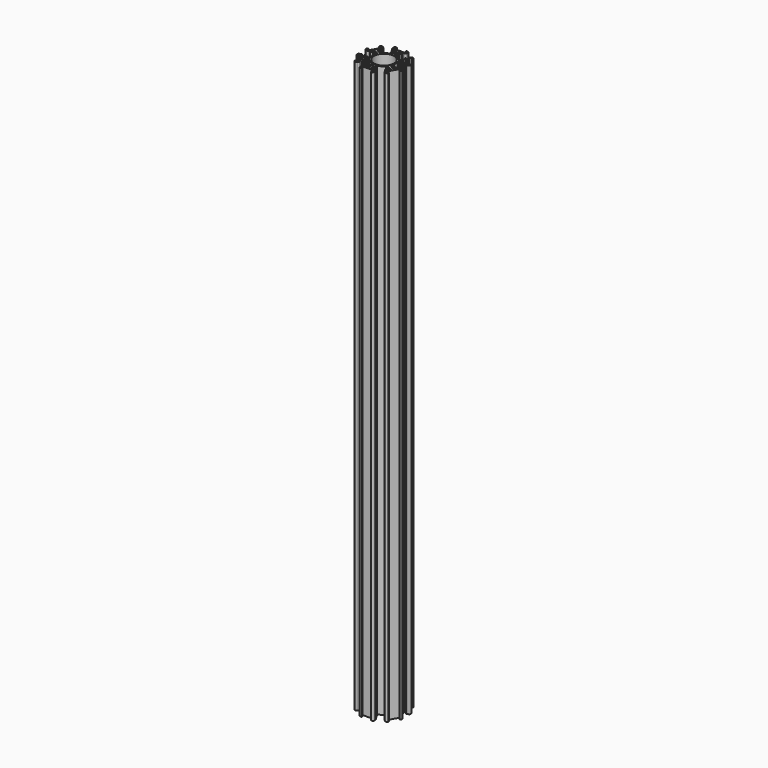
from build123d import *

# Parameters (mm, degrees)
F0_R     = 10.5
F1_DEPTH = 600
F2_R     = 1.5
F3_R     = 0.49999
F4_R     = 0.5
F6_DEPTH = 600.001
F7_R     = 0.5
F8_R     = 1.5


# Not quite as in the source:
# - a fillet or chamfer is up to 0.001 mm smaller than in the source, because OpenCascade refuses the exact size


with BuildPart() as f1:
    # F0 (on Top) → F1 (new body)
    with BuildSketch(Plane.XY):
        with BuildLine():
            Line((-7.45, -19.1599357944), (-7.45, -23.5599357944))
            Line((-7.45, -23.5599357944), (-4.75, -23.5599357944))
            Line((-4.75, -23.5599357944), (-4.75, -22.3599357944))
            Line((-4.75, -22.3599357944), (-6.25, -22.3599357944))
            Line((-6.25, -22.3599357944), (-6.25, -20.3599357944))
            Line((-6.25, -20.3599357944), (6.25, -20.3599357944))
            Line((6.25, -20.3599357944), (6.25, -22.3599357944))
            Line((6.25, -22.3599357944), (4.75, -22.3599357944))
            Line((4.75, -22.3599357944), (4.75, -23.5599357944))
            Line((4.75, -23.5599357944), (7.45, -23.5599357944))
            Line((7.45, -23.5599357944), (7.45, -19.1599357944))
            Line((7.45, -19.1599357944), (1, -19.1599357944))
            Line((1, -19.1599357944), (1, -17.4599357944))
            Line((1, -17.4599357944), (5.5, -17.4599357944))
            Line((5.5, -17.4599357944), (5.5, -16.4599357944))
            Line((5.5, -16.4599357944), (1, -16.4599357944))
            Line((1, -16.4599357944), (1, -14.8599357944))
            Line((1, -14.8599357944), (4, -14.8599357944))
            Line((4, -14.8599357944), (4, -13.8599357944))
            Line((4, -13.8599357944), (1, -13.8599357944))
            Line((1, -13.8599357944), (1, -12.4599357944))
            ThreePointArc((1, -12.4599357944), (6.25, -10.8253175473), (10.2906209275, -7.095993301))
            Line((10.2906209275, -7.095993301), (11.5030564928, -7.795993301))
            Line((11.5030564928, -7.795993301), (10.0030564928, -10.3940695123))
            Line((10.0030564928, -10.3940695123), (10.8690818965, -10.8940695123))
            Line((10.8690818965, -10.8940695123), (12.3690818965, -8.295993301))
            Line((12.3690818965, -8.295993301), (13.7547225426, -9.095993301))
            Line((13.7547225426, -9.095993301), (11.5047225426, -12.993107618))
            Line((11.5047225426, -12.993107618), (12.3707479464, -13.493107618))
            Line((12.3707479464, -13.493107618), (14.6207479464, -9.595993301))
            Line((14.6207479464, -9.595993301), (16.0929911328, -10.445993301))
            Line((16.0929911328, -10.445993301), (12.8679911328, -16.0318571554))
            Line((12.8679911328, -16.0318571554), (16.6785029095, -18.2318571554))
            Line((16.6785029095, -18.2318571554), (18.0285029095, -15.8935885652))
            Line((18.0285029095, -15.8935885652), (16.9892724249, -15.2935885652))
            Line((16.9892724249, -15.2935885652), (16.2392724249, -16.5926266708))
            Line((16.2392724249, -16.5926266708), (14.5072216174, -15.5926266708))
            Line((14.5072216174, -15.5926266708), (20.7572216174, -4.7673091235))
            Line((20.7572216174, -4.7673091235), (22.4892724249, -5.7673091235))
            Line((22.4892724249, -5.7673091235), (21.7392724249, -7.0663472292))
            Line((21.7392724249, -7.0663472292), (22.7785029095, -7.6663472292))
            Line((22.7785029095, -7.6663472292), (24.1285029095, -5.328078639))
            Line((24.1285029095, -5.328078639), (20.3179911328, -3.128078639))
            Line((20.3179911328, -3.128078639), (17.0929911328, -8.7139424934))
            Line((17.0929911328, -8.7139424934), (15.6207479464, -7.8639424934))
            Line((15.6207479464, -7.8639424934), (17.8707479464, -3.9668281764))
            Line((17.8707479464, -3.9668281764), (17.0047225426, -3.4668281764))
            Line((17.0047225426, -3.4668281764), (14.7547225426, -7.3639424934))
            Line((14.7547225426, -7.3639424934), (13.3690818965, -6.5639424934))
            Line((13.3690818965, -6.5639424934), (14.8690818965, -3.9658662821))
            Line((14.8690818965, -3.9658662821), (14.0030564928, -3.4658662821))
            Line((14.0030564928, -3.4658662821), (12.5030564928, -6.0639424934))
            Line((12.5030564928, -6.0639424934), (11.2906209275, -5.3639424934))
            ThreePointArc((11.2906209275, -5.3639424934), (12.5, 0), (11.2906209275, 5.3639424934))
            Line((11.2906209275, 5.3639424934), (12.5030564928, 6.0639424934))
            Line((12.5030564928, 6.0639424934), (14.0030564928, 3.4658662821))
            Line((14.0030564928, 3.4658662821), (14.8690818965, 3.9658662821))
            Line((14.8690818965, 3.9658662821), (13.3690818965, 6.5639424934))
            Line((13.3690818965, 6.5639424934), (14.7547225426, 7.3639424934))
            Line((14.7547225426, 7.3639424934), (17.0047225426, 3.4668281764))
            Line((17.0047225426, 3.4668281764), (17.8707479464, 3.9668281764))
            Line((17.8707479464, 3.9668281764), (15.6207479464, 7.8639424934))
            Line((15.6207479464, 7.8639424934), (17.0929911328, 8.7139424934))
            Line((17.0929911328, 8.7139424934), (20.3179911328, 3.128078639))
            Line((20.3179911328, 3.128078639), (24.1285029095, 5.328078639))
            Line((24.1285029095, 5.328078639), (22.7785029095, 7.6663472292))
            Line((22.7785029095, 7.6663472292), (21.7392724249, 7.0663472292))
            Line((21.7392724249, 7.0663472292), (22.4892724249, 5.7673091235))
            Line((22.4892724249, 5.7673091235), (20.7572216174, 4.7673091235))
            Line((20.7572216174, 4.7673091235), (14.5072216174, 15.5926266708))
            Line((14.5072216174, 15.5926266708), (16.2392724249, 16.5926266708))
            Line((16.2392724249, 16.5926266708), (16.9892724249, 15.2935885652))
            Line((16.9892724249, 15.2935885652), (18.0285029095, 15.8935885652))
            Line((18.0285029095, 15.8935885652), (16.6785029095, 18.2318571554))
            Line((16.6785029095, 18.2318571554), (12.8679911328, 16.0318571554))
            Line((12.8679911328, 16.0318571554), (16.0929911328, 10.445993301))
            Line((16.0929911328, 10.445993301), (14.6207479464, 9.595993301))
            Line((14.6207479464, 9.595993301), (12.3707479464, 13.493107618))
            Line((12.3707479464, 13.493107618), (11.5047225426, 12.993107618))
            Line((11.5047225426, 12.993107618), (13.7547225426, 9.095993301))
            Line((13.7547225426, 9.095993301), (12.3690818965, 8.295993301))
            Line((12.3690818965, 8.295993301), (10.8690818965, 10.8940695123))
            Line((10.8690818965, 10.8940695123), (10.0030564928, 10.3940695123))
            Line((10.0030564928, 10.3940695123), (11.5030564928, 7.795993301))
            Line((11.5030564928, 7.795993301), (10.2906209275, 7.095993301))
            ThreePointArc((10.2906209275, 7.095993301), (6.25, 10.8253175473), (1, 12.4599357944))
            Line((1, 12.4599357944), (1, 13.8599357944))
            Line((1, 13.8599357944), (4, 13.8599357944))
            Line((4, 13.8599357944), (4, 14.8599357944))
            Line((4, 14.8599357944), (1, 14.8599357944))
            Line((1, 14.8599357944), (1, 16.4599357944))
            Line((1, 16.4599357944), (5.5, 16.4599357944))
            Line((5.5, 16.4599357944), (5.5, 17.4599357944))
            Line((5.5, 17.4599357944), (1, 17.4599357944))
            Line((1, 17.4599357944), (1, 19.1599357944))
            Line((1, 19.1599357944), (7.45, 19.1599357944))
            Line((7.45, 19.1599357944), (7.45, 23.5599357944))
            Line((7.45, 23.5599357944), (4.75, 23.5599357944))
            Line((4.75, 23.5599357944), (4.75, 22.3599357944))
            Line((4.75, 22.3599357944), (6.25, 22.3599357944))
            Line((6.25, 22.3599357944), (6.25, 20.3599357944))
            Line((6.25, 20.3599357944), (-6.25, 20.3599357944))
            Line((-6.25, 20.3599357944), (-6.25, 22.3599357944))
            Line((-6.25, 22.3599357944), (-4.75, 22.3599357944))
            Line((-4.75, 22.3599357944), (-4.75, 23.5599357944))
            Line((-4.75, 23.5599357944), (-7.45, 23.5599357944))
            Line((-7.45, 23.5599357944), (-7.45, 19.1599357944))
            Line((-7.45, 19.1599357944), (-1, 19.1599357944))
            Line((-1, 19.1599357944), (-1, 17.4599357944))
            Line((-1, 17.4599357944), (-5.5, 17.4599357944))
            Line((-5.5, 17.4599357944), (-5.5, 16.4599357944))
            Line((-5.5, 16.4599357944), (-1, 16.4599357944))
            Line((-1, 16.4599357944), (-1, 14.8599357944))
            Line((-1, 14.8599357944), (-4, 14.8599357944))
            Line((-4, 14.8599357944), (-4, 13.8599357944))
            Line((-4, 13.8599357944), (-1, 13.8599357944))
            Line((-1, 13.8599357944), (-1, 12.4599357944))
            ThreePointArc((-1, 12.4599357944), (-6.25, 10.8253175473), (-10.2906209275, 7.095993301))
            Line((-10.2906209275, 7.095993301), (-11.5030564928, 7.795993301))
            Line((-11.5030564928, 7.795993301), (-10.0030564928, 10.3940695123))
            Line((-10.0030564928, 10.3940695123), (-10.8690818965, 10.8940695123))
            Line((-10.8690818965, 10.8940695123), (-12.3690818965, 8.295993301))
            Line((-12.3690818965, 8.295993301), (-13.7547225426, 9.095993301))
            Line((-13.7547225426, 9.095993301), (-11.5047225426, 12.993107618))
            Line((-11.5047225426, 12.993107618), (-12.3707479464, 13.493107618))
            Line((-12.3707479464, 13.493107618), (-14.6207479464, 9.595993301))
            Line((-14.6207479464, 9.595993301), (-16.0929911328, 10.445993301))
            Line((-16.0929911328, 10.445993301), (-12.8679911328, 16.0318571554))
            Line((-12.8679911328, 16.0318571554), (-16.6785029095, 18.2318571554))
            Line((-16.6785029095, 18.2318571554), (-18.0285029095, 15.8935885652))
            Line((-18.0285029095, 15.8935885652), (-16.9892724249, 15.2935885652))
            Line((-16.9892724249, 15.2935885652), (-16.2392724249, 16.5926266708))
            Line((-16.2392724249, 16.5926266708), (-14.5072216174, 15.5926266708))
            Line((-14.5072216174, 15.5926266708), (-20.7572216174, 4.7673091235))
            Line((-20.7572216174, 4.7673091235), (-22.4892724249, 5.7673091235))
            Line((-22.4892724249, 5.7673091235), (-21.7392724249, 7.0663472292))
            Line((-21.7392724249, 7.0663472292), (-22.7785029095, 7.6663472292))
            Line((-22.7785029095, 7.6663472292), (-24.1285029095, 5.328078639))
            Line((-24.1285029095, 5.328078639), (-20.3179911328, 3.128078639))
            Line((-20.3179911328, 3.128078639), (-17.0929911328, 8.7139424934))
            Line((-17.0929911328, 8.7139424934), (-15.6207479464, 7.8639424934))
            Line((-15.6207479464, 7.8639424934), (-17.8707479464, 3.9668281764))
            Line((-17.8707479464, 3.9668281764), (-17.0047225426, 3.4668281764))
            Line((-17.0047225426, 3.4668281764), (-14.7547225426, 7.3639424934))
            Line((-14.7547225426, 7.3639424934), (-13.3690818965, 6.5639424934))
            Line((-13.3690818965, 6.5639424934), (-14.8690818965, 3.9658662821))
            Line((-14.8690818965, 3.9658662821), (-14.0030564928, 3.4658662821))
            Line((-14.0030564928, 3.4658662821), (-12.5030564928, 6.0639424934))
            Line((-12.5030564928, 6.0639424934), (-11.2906209275, 5.3639424934))
            ThreePointArc((-11.2906209275, 5.3639424934), (-12.5, 0), (-11.2906209275, -5.3639424934))
            Line((-11.2906209275, -5.3639424934), (-12.5030564928, -6.0639424934))
            Line((-12.5030564928, -6.0639424934), (-14.0030564928, -3.4658662821))
            Line((-14.0030564928, -3.4658662821), (-14.8690818965, -3.9658662821))
            Line((-14.8690818965, -3.9658662821), (-13.3690818965, -6.5639424934))
            Line((-13.3690818965, -6.5639424934), (-14.7547225426, -7.3639424934))
            Line((-14.7547225426, -7.3639424934), (-17.0047225426, -3.4668281764))
            Line((-17.0047225426, -3.4668281764), (-17.8707479464, -3.9668281764))
            Line((-17.8707479464, -3.9668281764), (-15.6207479464, -7.8639424934))
            Line((-15.6207479464, -7.8639424934), (-17.0929911328, -8.7139424934))
            Line((-17.0929911328, -8.7139424934), (-20.3179911328, -3.128078639))
            Line((-20.3179911328, -3.128078639), (-24.1285029095, -5.328078639))
            Line((-24.1285029095, -5.328078639), (-22.7785029095, -7.6663472292))
            Line((-22.7785029095, -7.6663472292), (-21.7392724249, -7.0663472292))
            Line((-21.7392724249, -7.0663472292), (-22.4892724249, -5.7673091235))
            Line((-22.4892724249, -5.7673091235), (-20.7572216174, -4.7673091235))
            Line((-20.7572216174, -4.7673091235), (-14.5072216174, -15.5926266708))
            Line((-14.5072216174, -15.5926266708), (-16.2392724249, -16.5926266708))
            Line((-16.2392724249, -16.5926266708), (-16.9892724249, -15.2935885652))
            Line((-16.9892724249, -15.2935885652), (-18.0285029095, -15.8935885652))
            Line((-18.0285029095, -15.8935885652), (-16.6785029095, -18.2318571554))
            Line((-16.6785029095, -18.2318571554), (-12.8679911328, -16.0318571554))
            Line((-12.8679911328, -16.0318571554), (-16.0929911328, -10.445993301))
            Line((-16.0929911328, -10.445993301), (-14.6207479464, -9.595993301))
            Line((-14.6207479464, -9.595993301), (-12.3707479464, -13.493107618))
            Line((-12.3707479464, -13.493107618), (-11.5047225426, -12.993107618))
            Line((-11.5047225426, -12.993107618), (-13.7547225426, -9.095993301))
            Line((-13.7547225426, -9.095993301), (-12.3690818965, -8.295993301))
            Line((-12.3690818965, -8.295993301), (-10.8690818965, -10.8940695123))
            Line((-10.8690818965, -10.8940695123), (-10.0030564928, -10.3940695123))
            Line((-10.0030564928, -10.3940695123), (-11.5030564928, -7.795993301))
            Line((-11.5030564928, -7.795993301), (-10.2906209275, -7.095993301))
            ThreePointArc((-10.2906209275, -7.095993301), (-6.25, -10.8253175473), (-1, -12.4599357944))
            Line((-1, -12.4599357944), (-1, -13.8599357944))
            Line((-1, -13.8599357944), (-4, -13.8599357944))
            Line((-4, -13.8599357944), (-4, -14.8599357944))
            Line((-4, -14.8599357944), (-1, -14.8599357944))
            Line((-1, -14.8599357944), (-1, -16.4599357944))
            Line((-1, -16.4599357944), (-5.5, -16.4599357944))
            Line((-5.5, -16.4599357944), (-5.5, -17.4599357944))
            Line((-5.5, -17.4599357944), (-1, -17.4599357944))
            Line((-1, -17.4599357944), (-1, -19.1599357944))
            Line((-1, -19.1599357944), (-7.45, -19.1599357944))
        make_face()
        Circle(F0_R, mode=Mode.SUBTRACT)
    extrude(amount=F1_DEPTH)

    # F2
    f2_edges = [f1.edges().sort_by_distance(p)[0] for p in [
        (7.45, 19.159936, 300),
        (-7.45, 19.159936, 300),
        (12.867991, 16.031857, 300),
        (20.317991, 3.128079, 300),
        (20.317991, -3.128079, 300),
        (12.867991, -16.031857, 300),
        (7.45, -19.159936, 300),
        (-7.45, -19.159936, 300),
        (-12.867991, -16.031857, 300),
        (-20.317991, -3.128079, 300),
        (-20.317991, 3.128079, 300),
        (-12.867991, 16.031857, 300),
    ]]
    fillet(f2_edges, radius=F2_R)

    # F3 (radius 0.5 in the source; OpenCascade refuses exactly that, so slightly less here)
    f3_edges = [f1.edges().sort_by_distance(p)[0] for p in [
        (4.75, 23.559936, 300),
        (-4.75, 23.559936, 300),
        (-5.5, 17.459936, 300),
        (-5.5, 16.459936, 300),
        (-4, 14.859936, 300),
        (-4, 13.859936, 300),
        (5.5, 17.459936, 300),
        (5.5, 16.459936, 300),
        (4, 14.859936, 300),
        (4, 13.859936, 300),
        (-18.028503, 15.893589, 300),
        (-22.778503, 7.666347, 300),
        (-17.870748, 3.966828, 300),
        (-17.004723, 3.466828, 300),
        (-14.869082, 3.965866, 300),
        (-14.003056, 3.465866, 300),
        (-10.869082, 10.89407, 300),
        (-12.370748, 13.493108, 300),
        (-11.504723, 12.993108, 300),
        (-10.003056, 10.39407, 300),
        (-22.778503, -7.666347, 300),
        (-17.870748, -3.966828, 300),
        (-17.004723, -3.466828, 300),
        (-14.869082, -3.965866, 300),
        (-14.003056, -3.465866, 300),
        (-10.869082, -10.89407, 300),
        (-10.003056, -10.39407, 300),
        (-11.504723, -12.993108, 300),
        (-12.370748, -13.493108, 300),
        (-18.028503, -15.893589, 300),
        (-5.5, -17.459936, 300),
        (-5.5, -16.459936, 300),
        (-4, -14.859936, 300),
        (-4, -13.859936, 300),
        (-4.75, -23.559936, 300),
        (4.75, -23.559936, 300),
        (5.5, -17.459936, 300),
        (5.5, -16.459936, 300),
        (4, -14.859936, 300),
        (4, -13.859936, 300),
        (12.370748, -13.493108, 300),
        (11.504723, -12.993108, 300),
        (10.003056, -10.39407, 300),
        (10.869082, -10.89407, 300),
        (18.028503, -15.893589, 300),
        (22.778503, -7.666347, 300),
        (17.870748, -3.966828, 300),
        (14.869082, -3.965866, 300),
        (17.004723, -3.466828, 300),
        (14.003056, -3.465866, 300),
        (17.004723, 3.466828, 300),
        (17.870748, 3.966828, 300),
        (14.869082, 3.965866, 300),
        (14.003056, 3.465866, 300),
        (10.003056, 10.39407, 300),
        (11.504723, 12.993108, 300),
        (18.028503, 15.893589, 300),
        (22.778503, 7.666347, 300),
        (12.370748, 13.493108, 300),
        (10.869082, 10.89407, 300),
    ]]
    fillet(f3_edges, radius=F3_R)

    # F4
    f4_edges = [f1.edges().sort_by_distance(p)[0] for p in [
        (16.092991, -10.445993, 300),
        (17.092991, -8.713942, 300),
        (-1, -19.159936, 300),
        (1, -19.159936, 300),
        (-16.092991, -10.445993, 300),
        (-17.092991, -8.713942, 300),
        (-17.092991, 8.713942, 300),
        (-16.092991, 10.445993, 300),
        (-1, 19.159936, 300),
        (1, 19.159936, 300),
        (16.092991, 10.445993, 300),
        (17.092991, 8.713942, 300),
    ]]
    fillet(f4_edges, radius=F4_R)

    # F5 (on face) → F6 (cut, through all)
    with BuildSketch(Plane.XY.offset(600)):
        with BuildLine():
            Line((-1, 11.9582604777), (-1, 12.4599357944))
            ThreePointArc((-1, 12.4599357944), (-6.25, 10.8253175473), (-10.2906209275, 7.095993301))
            Line((-10.2906209275, 7.095993301), (-9.8561573587, 6.8451556426))
            ThreePointArc((-9.8561573587, 6.8451556426), (-5.9999998677, 10.3923046163), (-1, 11.9582604777))
        make_face()
        with BuildLine():
            Line((-10.8561575886, 5.1131049678), (-11.2906209275, 5.3639424934))
            ThreePointArc((-11.2906209275, 5.3639424934), (-12.5, 0), (-11.2906209275, -5.3639424934))
            Line((-11.2906209275, -5.3639424934), (-10.8561575886, -5.1131049678))
            ThreePointArc((-10.8561575886, -5.1131049678), (-12, 0), (-10.8561575886, 5.1131049678))
        make_face()
        with BuildLine():
            Line((-9.8561575886, -6.8451557753), (-10.2906209275, -7.095993301))
            ThreePointArc((-10.2906209275, -7.095993301), (-6.25, -10.8253175473), (-1, -12.4599357944))
            Line((-1, -12.4599357944), (-1, -11.9582607431))
            ThreePointArc((-1, -11.9582607431), (-6, -10.3923048454), (-9.8561575886, -6.8451557753))
        make_face()
        with BuildLine():
            Line((1, -11.9582604777), (1, -12.4599357944))
            ThreePointArc((1, -12.4599357944), (6.25, -10.8253175473), (10.2906209275, -7.095993301))
            Line((10.2906209275, -7.095993301), (9.8561573587, -6.8451556426))
            ThreePointArc((9.8561573587, -6.8451556426), (5.9999998677, -10.3923046163), (1, -11.9582604777))
        make_face()
        with BuildLine():
            Line((10.8561575886, -5.1131049678), (11.2906209275, -5.3639424934))
            ThreePointArc((11.2906209275, -5.3639424934), (12.5, 0), (11.2906209275, 5.3639424934))
            Line((11.2906209275, 5.3639424934), (10.8561575886, 5.1131049678))
            ThreePointArc((10.8561575886, 5.1131049678), (12, 0), (10.8561575886, -5.1131049678))
        make_face()
        with BuildLine():
            Line((9.8561573587, 6.8451556426), (10.2906209275, 7.095993301))
            ThreePointArc((10.2906209275, 7.095993301), (6.25, 10.8253175473), (1, 12.4599357944))
            Line((1, 12.4599357944), (1, 11.9582604777))
            ThreePointArc((1, 11.9582604777), (5.9999998677, 10.3923046163), (9.8561573587, 6.8451556426))
        make_face()
    extrude(amount=-F6_DEPTH, mode=Mode.SUBTRACT)

    # F7
    f7_edges = [f1.edges().sort_by_distance(p)[0] for p in [
        (21.739272, -7.066347, 300),
        (16.989272, -15.293589, 300),
        (4.75, -22.359936, 300),
        (-4.75, -22.359936, 300),
        (-16.989272, -15.293589, 300),
        (-21.739272, -7.066347, 300),
        (-21.739272, 7.066347, 300),
        (-16.989272, 15.293589, 300),
        (-4.75, 22.359936, 300),
        (4.75, 22.359936, 300),
        (16.989272, 15.293589, 300),
        (21.739272, 7.066347, 300),
        (-9.856158, -6.845156, 300),
        (-10.856158, -5.113105, 300),
        (-10.856158, 5.113105, 300),
        (-9.856157, 6.845156, 300),
        (-1, 11.95826, 300),
        (1, 11.95826, 300),
        (9.856157, 6.845156, 300),
        (10.856158, 5.113105, 300),
        (10.856158, -5.113105, 300),
        (9.856157, -6.845156, 300),
        (1, -11.95826, 300),
        (-1, -11.958261, 300),
    ]]
    fillet(f7_edges, radius=F7_R)

    # F8
    f8_edges = [f1.edges().sort_by_distance(p)[0] for p in [
        (24.128503, -5.328079, 300),
        (16.678503, -18.231857, 300),
        (24.128503, 5.328079, 300),
        (16.678503, 18.231857, 300),
        (7.45, 23.559936, 300),
        (-7.45, 23.559936, 300),
        (-16.678503, 18.231857, 300),
        (-24.128503, 5.328079, 300),
        (-24.128503, -5.328079, 300),
        (-16.678503, -18.231857, 300),
        (-7.45, -23.559936, 300),
        (7.45, -23.559936, 300),
    ]]
    fillet(f8_edges, radius=F8_R)


solid = f1.part
